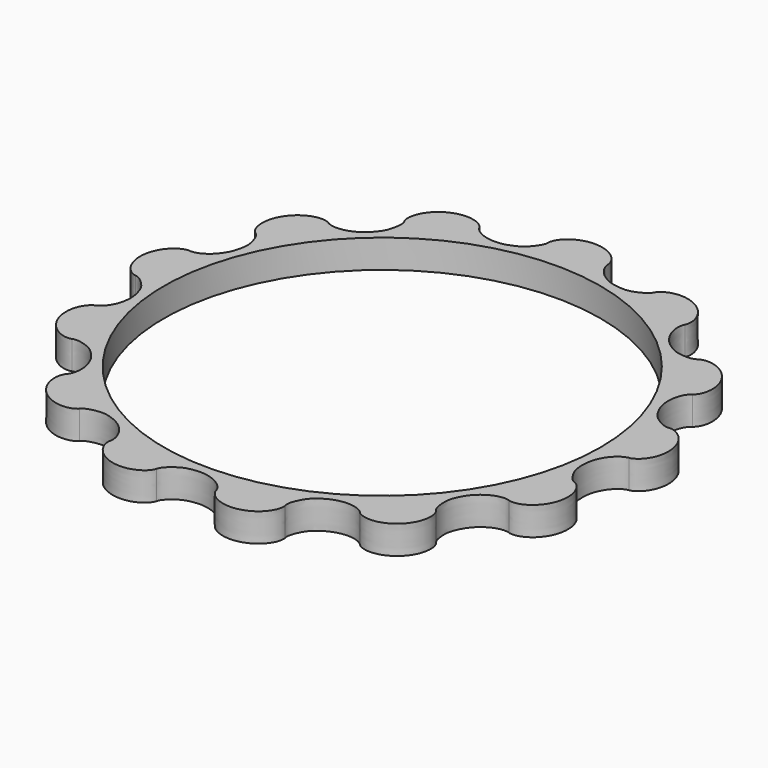
from build123d import *

# Parameters (mm, degrees)
F1_R            = 26
F2_DEPTH        = 3
F4_DEPTH        = 3
F4_COPIES_COUNT = 13
F6_DEPTH        = 3.0010001
F6_COPIES_COUNT = 13
F7_R            = 23
F8_DEPTH        = 3.0010001


# Not quite as in the source:
# - a pattern or mirror of a feature is missing from the dataset's text; its kind, count and spacing are read off the source's solid


with BuildPart() as f2:
    # F1 (on Top) → F2 (new body)
    with BuildSketch(Plane.XY):
        Circle(F1_R)
    extrude(amount=F2_DEPTH)

    # F3 (on face) → F4 (join, through all)
    with BuildSketch(Plane.XY.offset(3)):
        with BuildLine():
            add(Edge.make_bspline(
                [(25.2444872531, 6.2222072715), (25.2930343439, 6.2341730547), (25.3914485115, 6.2353621958), (25.8307327393, 6.1683615414), (26.4089164088, 5.8694283629), (27.048033967, 5.2848705912), (27.5669226238, 4.4237892835), (27.8467853727, 3.3812103206), (27.8245598182, 2.3019546028), (27.5268195126, 1.3417161773), (27.0461677041, 0.6211940302), (26.5563233447, 0.1925786095), (26.1458436624, 0.0223990485), (26.0499999753, 0), (26, 4.96544e-05)],
                knots=[0, 0, 0, 0, 0.0392234913, 0.1063514424, 0.1910137456, 0.2876622776, 0.3919583336, 0.5000007182, 0.6080429525, 0.7123390084, 0.8089875404, 0.8936498436, 0.9607777947, 1, 1, 1, 1], degree=3))
            ThreePointArc((25.2444872531, 6.2222072715), (25.3058591438, 5.9677041646), (25.364665322, 5.7125960037))
            ThreePointArc((25.364665322, 5.7125960037), (25.4208998256, 5.4569086537), (25.4745569531, 5.2006680382))
            ThreePointArc((25.4745569531, 5.2006680382), (25.8683032159, 2.6135968948), (26, 4.96544e-05))
        make_face()
        with BuildLine():
            add(Edge.make_bspline(
                [(2.4619489833, 3.0403513771), (2.5104960742, 3.0523171603), (2.6285965776, 2.9347604264), (3.0814324081, 2.837058921), (3.6772292572, 2.4487691881), (4.3287147738, 1.7936826337), (4.8595203047, 0.8548336965), (5.1494923728, -0.2641289718), (5.1355418512, -1.419863584), (4.8457093071, -2.4587293971), (4.3670103699, -3.2498319559), (3.8902992691, -3.7720193929), (3.4562341665, -3.9662691802), (3.4043836091, -4.1157155272), (3.354383646, -4.1156547643)],
                knots=[0, 0, 0, 0, 0.0417531183, 0.1090741669, 0.1935200595, 0.2897789734, 0.3935965528, 0.5011209261, 0.608645347, 0.7124629265, 0.8087218404, 0.893167733, 0.9604887816, 1, 1, 1, 1], degree=3))
            ThreePointArc((2.4619489833, 3.0403513771), (3.1239697933, -0.5107385662), (3.354383646, -4.1156547643))
        make_face()
    f4 = extrude(amount=-F4_DEPTH)

    # F4_copies: F4 ×13 about axis
    f4_copies_axis = Axis((0, 0, 0), (0, 0, 1))
    for i in range(1, F4_COPIES_COUNT):
        add(f4.rotate(f4_copies_axis, i * 360 / F4_COPIES_COUNT))

    # F5 (on face) → F6 (cut, through all)
    with BuildSketch(Plane.XY.offset(3)):
        with BuildLine():
            ThreePointArc((23.2605005387, 11.616760077), (23.1423517821, 11.8503820188), (23.021856667, 12.0828024731))
            add(Edge.make_bspline(
                [(25.2444872531, 6.2222072715), (25.1959401622, 6.2102414883), (25.1034931503, 6.2132271636), (24.6779908905, 6.2070613183), (23.428636921, 6.9001908976), (22.895177954, 7.6000880267), (22.3944218587, 8.4997532621), (22.1662851887, 9.4632576695), (22.1623780227, 10.3925790979), (22.3580005057, 11.1688899152), (22.6288188045, 11.7031177653), (22.9130532602, 12.0056360148), (22.9775838657, 12.0595663145), (23.021856667, 12.0828024731)],
                knots=[0, 0, 0, 0, 0.041425265, 0.1123306525, 0.247572754, 0.3577393511, 0.4718631356, 0.5859868742, 0.6961534713, 0.7982419786, 0.8876693475, 0.958574735, 1, 1, 1, 1], degree=3))
            ThreePointArc((25.2444872531, 6.2222072715), (24.4020236899, 8.9744771344), (23.2605005387, 11.616760077))
        make_face()
    f6 = extrude(amount=-F6_DEPTH, mode=Mode.SUBTRACT)

    # F6_copies: F6 ×13 about axis
    f6_copies_axis = Axis((0, 0, 0), (0, 0, 1))
    for i in range(1, F6_COPIES_COUNT):
        add(f6.rotate(f6_copies_axis, i * 360 / F6_COPIES_COUNT), mode=Mode.SUBTRACT)

    # F7 (on face) → F8 (cut, through all)
    with BuildSketch(Plane.XY.offset(3)):
        Circle(F7_R)
    extrude(amount=-F8_DEPTH, mode=Mode.SUBTRACT)


solid = f2.part
